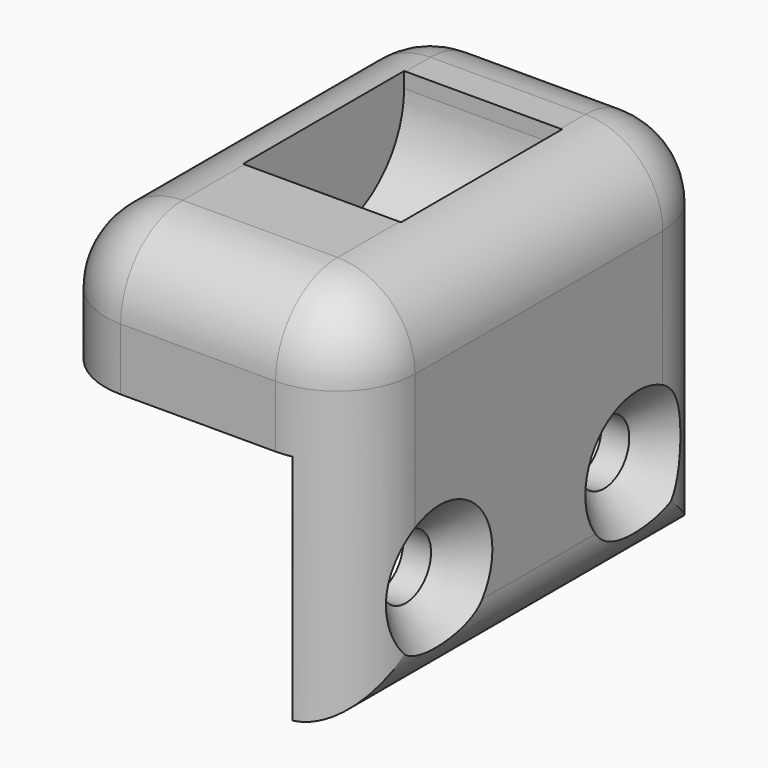
from build123d import *

# Parameters (mm, degrees)
F0_W            = 20
F0_H            = 30
F1_DEPTH        = 9
F4_W            = 10.2
F4_H            = 13
F5_DEPTH        = 7
F2_W            = 4
F2_H            = 30
F6_DEPTH        = 15
F7_R            = 6
F10_D           = 4.1
F10_CSINK_D     = 8.5
F10_CSINK_ANGLE = 90
F11_F1_R        = 5
F11_F2_R        = 5
F11_T3_DEPTH    = 20
F11_T5_DEPTH    = 16.5
F11_T8_ANGLE    = 90
F11_T10_ANGLE   = 90
F11_T11_DEPTH   = 20
F11_T13_DEPTH   = 31.5
F11_T16_ANGLE   = 90
F11_T18_ANGLE   = 90
F13_T1_DEPTH    = 40


# Not quite as in the source:
# - a fillet or chamfer that OpenCascade refuses, or shapes differently, is made with other operations: its cross-section is extruded or revolved along the edge and cut away or added
# - a feature of the source that left no trace in its solid (it failed there, or was rolled back) is left out


with BuildPart() as f1:
    # F0 (on Top) → F1 (new body)
    with BuildSketch(Plane.XY):
        with Locations((-10, 15)):
            Rectangle(F0_W, F0_H)
    extrude(amount=F1_DEPTH)

    # F4 (on offset) → F5 (cut)
    with BuildSketch(Plane.XY.offset(9)):
        with Locations((-10, 16.5)):
            Rectangle(F4_W, F4_H)
    extrude(amount=-F5_DEPTH, mode=Mode.SUBTRACT)

    # F2 (on Top) → F6 (join)
    with BuildSketch(Plane.XY):
        with Locations((-2, 15)):
            Rectangle(F2_W, F2_H)
    extrude(amount=-F6_DEPTH)

    # F7
    f7_edges = [f1.edges().sort_by_distance(p)[0] for p in [
        (-10, 10, 2),
        (-10, 23, 2),
    ]]
    fillet(f7_edges, radius=F7_R)

    # F10 (through all)
    with Locations(Plane.YZ):
        with Locations((7, -8.5), (23, -8.5)):
            CounterSinkHole(F10_D / 2, F10_CSINK_D / 2, counter_sink_angle=F10_CSINK_ANGLE)

    # F11: fillet of radius 5 on 4 edges, made by hand

    # F11_f1
    f11_f1_edges = [f1.edges().sort_by_distance(p)[0] for p in [
        (-10, 0, 9),
    ]]
    fillet(f11_f1_edges, radius=F11_F1_R)

    # F11_f2
    f11_f2_edges = [f1.edges().sort_by_distance(p)[0] for p in [
        (-10, 30, 9),
    ]]
    fillet(f11_f2_edges, radius=F11_F2_R)

    # F11_s4 → F11_t3 (cut)
    with BuildSketch(Plane.XZ.offset(-25)):
        with BuildLine():
            ThreePointArc((-15, 9), (-18.5355339059, 7.5355339059), (-20, 4))
            Line((-20, 4), (-20.1, 4))
            Line((-20.1, 4), (-20.1, 9.1))
            Line((-20.1, 9.1), (-15, 9.1))
            Line((-15, 9.1), (-15, 9))
        make_face()
    extrude(amount=F11_T3_DEPTH, mode=Mode.SUBTRACT)

    # F11_s6 → F11_t5 (cut)
    with BuildSketch(Plane.XY.offset(-12.5)):
        with BuildLine():
            ThreePointArc((-20, 5), (-18.5355339059, 1.4644660941), (-15, 0))
            Line((-15, 0), (-15, -0.1))
            Line((-15, -0.1), (-20.1, -0.1))
            Line((-20.1, -0.1), (-20.1, 5))
            Line((-20.1, 5), (-20, 5))
        make_face()
        with BuildLine():
            ThreePointArc((-20, 25), (-18.5355339059, 28.5355339059), (-15, 30))
            Line((-15, 30), (-15, 30.1))
            Line((-15, 30.1), (-20.1, 30.1))
            Line((-20.1, 30.1), (-20.1, 25))
            Line((-20.1, 25), (-20, 25))
        make_face()
    extrude(amount=F11_T5_DEPTH, mode=Mode.SUBTRACT)

    # F11_s7 → F11_t8 (revolve, cut)
    with BuildSketch(Plane.XZ.offset(-25)):
        with BuildLine():
            ThreePointArc((-20, 4), (-18.5355339059, 7.5355339059), (-15, 9))
            Line((-15, 9), (-15, 9.1))
            Line((-15, 9.1), (-20.1, 9.1))
            Line((-20.1, 9.1), (-20.1, 4))
            Line((-20.1, 4), (-20, 4))
        make_face()
    revolve(axis=Axis((-20, 25, 4), (-1, 0, 0)), revolution_arc=F11_T8_ANGLE, mode=Mode.SUBTRACT)

    # F11_s9 → F11_t10 (revolve, cut)
    with BuildSketch(Plane.XZ.offset(-5)):
        with BuildLine():
            ThreePointArc((-20, 4), (-18.5355339059, 7.5355339059), (-15, 9))
            Line((-15, 9), (-15, 9.1))
            Line((-15, 9.1), (-20.1, 9.1))
            Line((-20.1, 9.1), (-20.1, 4))
            Line((-20.1, 4), (-20, 4))
        make_face()
    revolve(axis=Axis((-20, 5, 4), (1, 0, 0)), revolution_arc=F11_T10_ANGLE, mode=Mode.SUBTRACT)

    # F11_s12 → F11_t11 (cut)
    with BuildSketch(Plane.XZ.offset(-25)):
        with BuildLine():
            ThreePointArc((-5, 9), (-1.4644660941, 7.5355339059), (0, 4))
            Line((0, 4), (0.1, 4))
            Line((0.1, 4), (0.1, 9.1))
            Line((0.1, 9.1), (-5, 9.1))
            Line((-5, 9.1), (-5, 9))
        make_face()
    extrude(amount=F11_T11_DEPTH, mode=Mode.SUBTRACT)

    # F11_s14 → F11_t13 (cut)
    with BuildSketch(Plane.XY.offset(-27.5)):
        with BuildLine():
            ThreePointArc((0, 25), (-1.4644660941, 28.5355339059), (-5, 30))
            Line((-5, 30), (-5, 30.1))
            Line((-5, 30.1), (0.1, 30.1))
            Line((0.1, 30.1), (0.1, 25))
            Line((0.1, 25), (0, 25))
        make_face()
        with BuildLine():
            ThreePointArc((0, 5), (-1.4644660941, 1.4644660941), (-5, 0))
            Line((-5, 0), (-5, -0.1))
            Line((-5, -0.1), (0.1, -0.1))
            Line((0.1, -0.1), (0.1, 5))
            Line((0.1, 5), (0, 5))
        make_face()
    extrude(amount=F11_T13_DEPTH, mode=Mode.SUBTRACT)

    # F11_s15 → F11_t16 (revolve, cut)
    with BuildSketch(Plane.XZ.offset(-5)):
        with BuildLine():
            ThreePointArc((0, 4), (-1.4644660941, 7.5355339059), (-5, 9))
            Line((-5, 9), (-5, 9.1))
            Line((-5, 9.1), (0.1, 9.1))
            Line((0.1, 9.1), (0.1, 4))
            Line((0.1, 4), (0, 4))
        make_face()
    revolve(axis=Axis((0, 5, 4), (1, 0, 0)), revolution_arc=F11_T16_ANGLE, mode=Mode.SUBTRACT)

    # F11_s17 → F11_t18 (revolve, cut)
    with BuildSketch(Plane.XZ.offset(-25)):
        with BuildLine():
            ThreePointArc((-5, 9), (-1.4644660941, 7.5355339059), (0, 4))
            Line((0, 4), (0.1, 4))
            Line((0.1, 4), (0.1, 9.1))
            Line((0.1, 9.1), (-5, 9.1))
            Line((-5, 9.1), (-5, 9))
        make_face()
    revolve(axis=Axis((0, 25, 4), (-1, 0, 0)), revolution_arc=F11_T18_ANGLE, mode=Mode.SUBTRACT)

    # F13: fillet of radius 4 on 1 edges, made by hand

    # F13_s2 → F13_t1 (cut)
    with BuildSketch(Plane.XZ.offset(-35)):
        with BuildLine():
            ThreePointArc((0, -11), (-1.1715728753, -13.8284271247), (-4, -15))
            Line((-4, -15), (0, -15))
            Line((0, -15), (0, -11))
        make_face()
    extrude(amount=F13_T1_DEPTH, mode=Mode.SUBTRACT)


solid = f1.part
